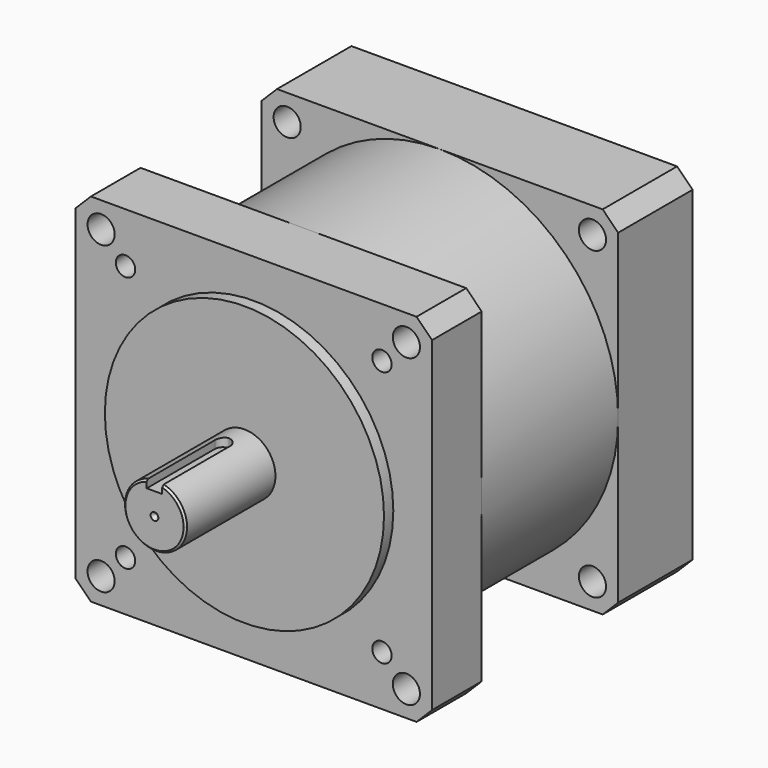
from build123d import *

# Parameters (mm, degrees)
F0_W      = 146.05
F0_H      = 146.05
F1_DEPTH  = 133.35
F2_DEPTH  = 107.95
F3_DEPTH  = 38.1
F4_R      = 73.025
F5_DEPTH  = 133.35
F6_D      = 11.1125
F8_D      = 6.5278
F8_DEPTH  = 25.4
F8_TIP    = 1.9611489744
F7_R      = 50.292
F7_R_2    = 19.05
F9_DEPTH  = 19.05
F7_R_3    = 54.991
F10_DEPTH = 6.35
F11_DEPTH = 101.6
F12_R     = 12.7
F13_DEPTH = 133.351
F12_R_2   = 57.15
F14_DEPTH = 4.7625
F15_D     = 7.9375
F15_DEPTH = 19.05
F15_TIP   = 2.3846655818
F16_SIZE  = 6.35
F17_DEPTH = 50.8
F19_DEPTH = 38.1
F20_R     = 3.1749
F18_R     = 1.5875
F21_DEPTH = 1.5875
F22_SIZE  = 1.58749
F23_SIZE  = 0.79375


# Not quite as in the source:
# - a fillet or chamfer is up to 0.001 mm smaller than in the source, because OpenCascade refuses the exact size
# - a length typed as a fraction of an inch, garbled in the dataset ("3 / 203.2 mm" for 3/8 in), is restored


with BuildPart() as f1:
    # F0 (on Front) → F1 (new body)
    with BuildSketch(Plane.XZ):
        Rectangle(F0_W, F0_H)
    extrude(amount=F1_DEPTH)

    # F2 (cut): a face of the model
    f2_faces = [f1.faces().sort_by_distance(p)[0] for p in [
        (0, 0, 0),
    ]]
    extrude(f2_faces, amount=-F2_DEPTH, mode=Mode.SUBTRACT)



with BuildPart() as f3:
    # F0 (on Front) → F3 (new body)
    with BuildSketch(Plane.XZ):
        Rectangle(F0_W, F0_H)
    extrude(amount=F3_DEPTH)


with BuildPart() as f1_1:
    add(f1.part)

    add(f3.part)  # F5 merges F3
    # F4 (on face) → F5 (join, through all)
    with BuildSketch(Plane.XZ):
        Circle(F4_R)
    extrude(amount=F5_DEPTH)

    # F6 (through all)
    with Locations(Plane(origin=(0, 0, 0), x_dir=(1, 0, 0), z_dir=(0, 1, 0))):
        with Locations((62.5, -62.5), (-62.5, -62.5), (-62.5, 62.5), (62.5, 62.5)):
            Hole(F6_D / 2)

    # F8
    with Locations(Plane(origin=(0, 0, 0), x_dir=(1, 0, 0), z_dir=(0, 1, 0))):
        with Locations((-45.72, -45.72), (45.72, -45.72), (45.72, 45.72), (-45.72, 45.72)):
            Hole(F8_D / 2, depth=F8_DEPTH)
            with Locations((0, 0, -(F8_DEPTH + F8_TIP / 2))):  # 118° drill point
                Cone(0, F8_D / 2, F8_TIP, mode=Mode.SUBTRACT)

    # F7 (on face) → F9 (cut)
    with BuildSketch(Plane.XZ):
        Circle(F7_R)
        Circle(F7_R_2, mode=Mode.SUBTRACT)
    extrude(amount=F9_DEPTH, mode=Mode.SUBTRACT)

    # F7 (on face) → F10 (cut)
    with BuildSketch(Plane.XZ):
        Circle(F7_R_3)
        Circle(F7_R, mode=Mode.SUBTRACT)
    extrude(amount=F10_DEPTH, mode=Mode.SUBTRACT)

    # F7 (on face) → F11 (cut)
    with BuildSketch(Plane.XZ):
        Circle(F7_R_2)
    extrude(amount=F11_DEPTH, mode=Mode.SUBTRACT)

    # F12 (on face) → F13 (cut, through all)
    with BuildSketch(Plane.XZ.offset(133.35)):
        Circle(F12_R)
    extrude(amount=-F13_DEPTH, mode=Mode.SUBTRACT)

    # F12 (on face) → F14 (join)
    with BuildSketch(Plane.XZ.offset(133.35)):
        Circle(F12_R_2)
        Circle(F12_R, mode=Mode.SUBTRACT)
    extrude(amount=F14_DEPTH)

    # F15
    with Locations(Plane.XZ.offset(133.35)):
        with Locations((52.5, 52.5018), (52.5, -52.4982), (-52.5, -52.4982), (-52.5, 52.5018)):
            Hole(F15_D / 2, depth=F15_DEPTH)
            with Locations((0, 0, -(F15_DEPTH + F15_TIP / 2))):  # 118° drill point
                Cone(0, F15_D / 2, F15_TIP, mode=Mode.SUBTRACT)

    # F16
    f16_edges = [f1_1.edges().sort_by_distance(p)[0] for p in [
        (73.025, -19.05, 73.025),
        (73.025, -120.65, 73.025),
        (73.025, -19.05, -73.025),
        (73.025, -120.65, -73.025),
        (-73.025, -19.05, -73.025),
        (-73.025, -120.65, -73.025),
        (-73.025, -19.05, 73.025),
        (-73.025, -120.65, 73.025),
    ]]
    chamfer(f16_edges, length=F16_SIZE)


with BuildPart() as f17:
    # F12 (on face) → F17 (new body)
    with BuildSketch(Plane.XZ.offset(133.35)):
        Circle(F12_R)
    extrude(amount=F17_DEPTH)

    # F18 (on face) → F19 (cut)
    with BuildSketch(Plane.XZ.offset(184.15)):
        with BuildLine():
            Line((-3.175, 9.1217221242), (0, 9.1217221242))
            Line((0, 9.1217221242), (3.175, 9.1217221242))
            Line((3.175, 9.1217221242), (3.175, 12.2967221242))
            ThreePointArc((3.175, 12.2967221242), (0, 12.7), (-3.175, 12.2967221242))
            Line((-3.175, 12.2967221242), (-3.175, 9.1217221242))
        make_face()
    extrude(amount=-F19_DEPTH, mode=Mode.SUBTRACT)

    # F20 (radius 3.175 in the source; OpenCascade refuses exactly that, so slightly less here)
    f20_edges = [f17.edges().sort_by_distance(p)[0] for p in [
        (-3.175, -146.05, 10.709222),
        (3.175, -146.05, 10.709222),
    ]]
    fillet(f20_edges, radius=F20_R)

    # F18 (on face) → F21 (cut)
    with BuildSketch(Plane.XZ.offset(184.15)):
        Circle(F18_R)
    extrude(amount=-F21_DEPTH, mode=Mode.SUBTRACT)

    # F22 (size 1.5875 in the source; OpenCascade refuses exactly that, so slightly less here)
    f22_edges = [f17.edges().sort_by_distance(p)[0] for p in [
        (-1.5875, -182.5625, 0),
    ]]
    chamfer(f22_edges, length=F22_SIZE)

    # F23
    f23_edges = [f17.edges().sort_by_distance(p)[0] for p in [
        (-7.77713, -184.15, -10.040232),
    ]]
    chamfer(f23_edges, length=F23_SIZE)


solid = Compound([f1_1.part, f17.part])
